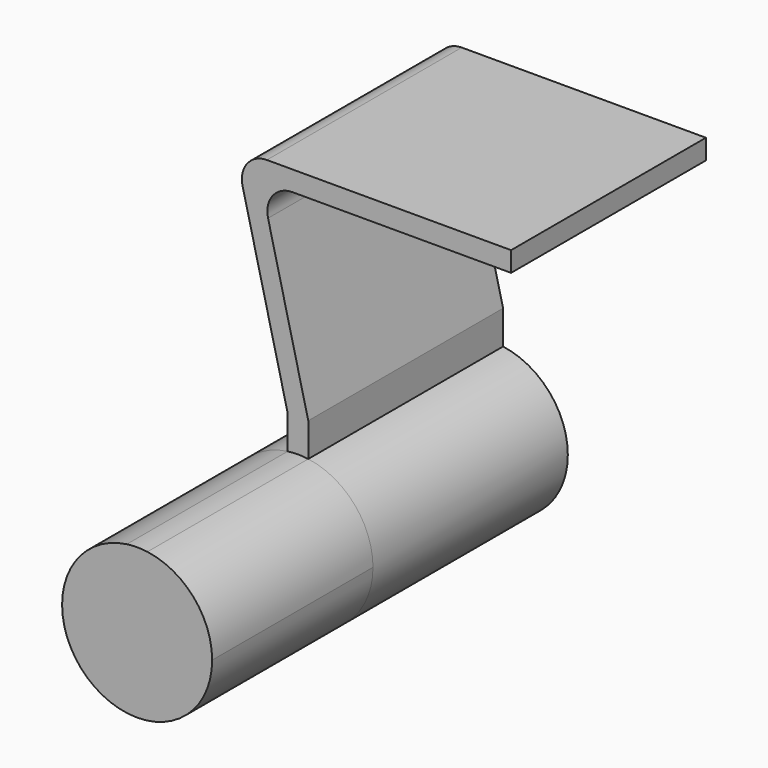
from build123d import *

# Parameters (mm, degrees)
F0_W      = 70.085093379
F0_H      = 61.8397891521
F1_DEPTH  = 54.864
F3_DEPTH  = 61.8407891521
F4_W      = 5.2283558833
F4_H      = 61.8397891521
F5_DEPTH  = 8.382
F6_W      = 5.2283558833
F6_H      = 61.8397891521
F6_W_2    = 16.4358220583
F7_DEPTH  = 38.1
F9_DEPTH  = 25.4
F10_DEPTH = 36.4407891521
F12_DEPTH = 51.054


# Not quite as in the source:
# - after a boolean that leaves OpenCascade's solid faulty, fix() repairs it


with BuildPart() as f1:
    # F0 (on Top) → F1 (new body)
    with BuildSketch(Plane.XY):
        with Locations((-35.0425466895, 30.9198945761)):
            Rectangle(F0_W, F0_H)
    extrude(amount=-F1_DEPTH)

    # F2 (on face) → F3 (cut, through all)
    with BuildSketch(Plane(origin=(0, 61.8397891521, 0), x_dir=(-1, 0, 0), z_dir=(0, 1, 0))):
        with BuildLine():
            Line((0, -54.864), (51.500908674, -54.864))
            Line((51.500908674, -54.864), (61.7086454928, -12.9319506824))
            ThreePointArc((61.7086454928, -12.9319506824), (60.5318177305, -7.5066651196), (55.5388283037, -5.08))
            Line((55.5388283037, -5.08), (52.6744276285, -5.08))
            Line((52.6744276285, -5.08), (0, -5.08))
            Line((0, -5.08), (0, -54.864))
        make_face()
        with BuildLine():
            ThreePointArc((62.0038350038, 0), (66.9968244307, -2.4266651196), (68.173652193, -7.8519506824))
            Line((68.173652193, -7.8519506824), (56.7292645574, -54.864))
            Line((56.7292645574, -54.864), (70.085093379, -54.864))
            Line((70.085093379, -54.864), (70.085093379, 0))
            Line((70.085093379, 0), (62.0038350038, 0))
        make_face()
    extrude(amount=-F3_DEPTH, mode=Mode.SUBTRACT)

    # F4 (on face) → F5 (join)
    with BuildSketch(Plane(origin=(0, 0, -54.864), x_dir=(1, 0, 0), z_dir=(0, 0, -1))):
        with Locations((-54.1150866157, -30.9198945761)):
            Rectangle(F4_W, F4_H)
    extrude(amount=F5_DEPTH)

    # F6 (on face) → F7 (join)
    with BuildSketch(Plane(origin=(0, 0, -63.246), x_dir=(1, 0, 0), z_dir=(0, 0, -1))):
        with Locations((-54.1150866157, -30.9198945761)):
            Rectangle(F6_W, F6_H)
        with Locations((-43.2829976449, -30.9198945761)):
            Rectangle(F6_W_2, F6_H)
        with Locations((-64.9471755865, -30.9198945761)):
            Rectangle(F6_W_2, F6_H)
    extrude(amount=F7_DEPTH)

    # F8 (on face) → F9 (cut)
    with BuildSketch(Plane.XZ):
        with BuildLine():
            ThreePointArc((-51.500908674, -63.4262206243), (-39.7501537967, -69.7839575966), (-35.0650866157, -82.296))
            Line((-35.0650866157, -82.296), (-35.0650866157, -63.246))
            Line((-35.0650866157, -63.246), (-51.500908674, -63.246))
            Line((-51.500908674, -63.246), (-51.500908674, -63.4262206243))
        make_face()
        with BuildLine():
            ThreePointArc((-73.1650866157, -82.296), (-68.4800194347, -69.7839575966), (-56.7292645574, -63.4262206243))
            Line((-56.7292645574, -63.4262206243), (-56.7292645574, -63.246))
            Line((-56.7292645574, -63.246), (-73.1650866157, -63.246))
            Line((-73.1650866157, -63.246), (-73.1650866157, -82.296))
        make_face()
        with BuildLine():
            Line((-35.0650866157, -101.346), (-35.0650866157, -82.296))
            ThreePointArc((-35.0650866157, -82.296), (-40.6447024341, -95.7663841816), (-54.1150866157, -101.346))
            Line((-54.1150866157, -101.346), (-35.0650866157, -101.346))
        make_face()
        with BuildLine():
            Line((-73.1650866157, -101.346), (-54.1150866157, -101.346))
            ThreePointArc((-54.1150866157, -101.346), (-67.5854707973, -95.7663841816), (-73.1650866157, -82.296))
            Line((-73.1650866157, -82.296), (-73.1650866157, -101.346))
        make_face()
    extrude(amount=-F9_DEPTH, mode=Mode.SUBTRACT)

    # F10 (cut, through all): faces of the model
    f10_faces = [f1.faces().sort_by_distance(p)[0] for p in [
        (-39.2943641898, 25.4, -67.5096317249),
        (-39.3202458526, 25.4, -97.0908407631),
        (-68.9099273788, 25.4, -97.0908407631),
        (-68.9358090416, 25.4, -67.5096317249),
    ]]
    extrude(f10_faces, amount=-F10_DEPTH, mode=Mode.SUBTRACT)

    # F11 (on face) → F12 (join)
    with BuildSketch(Plane.XZ):
        with BuildLine():
            ThreePointArc((-73.1650866157, -82.296), (-54.1150866157, -101.346), (-35.0650866157, -82.296))
            ThreePointArc((-35.0650866157, -82.296), (-39.7501537967, -69.7839575966), (-51.500908674, -63.4262206243))
            ThreePointArc((-51.500908674, -63.4262206243), (-54.1150866157, -63.246), (-56.7292645574, -63.4262206243))
            ThreePointArc((-56.7292645574, -63.4262206243), (-68.4800194347, -69.7839575966), (-73.1650866157, -82.296))
        make_face()
    extrude(amount=F12_DEPTH)

    add(f1.part.fix(), mode=Mode.REPLACE)


solid = f1.part
